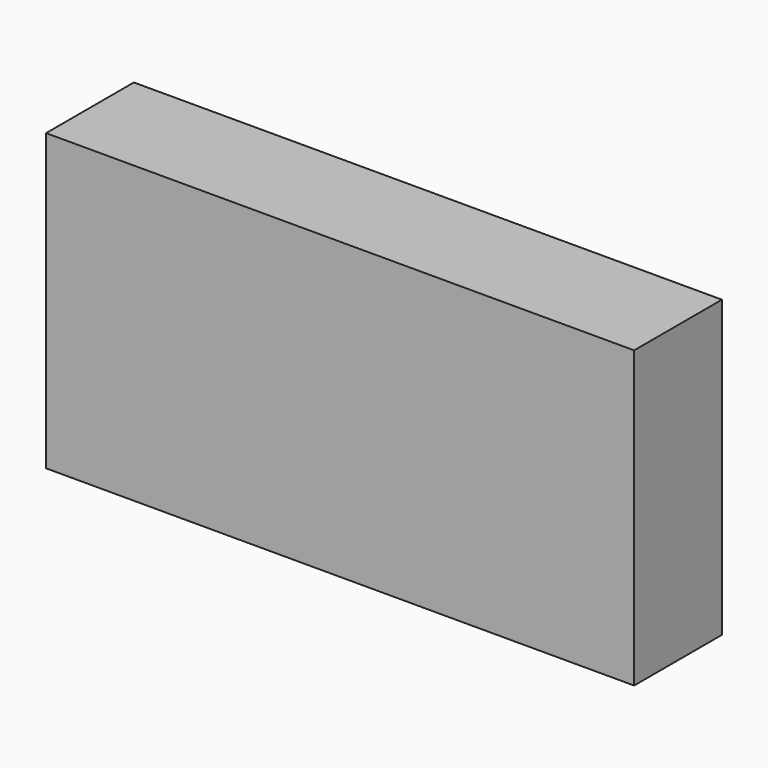
from build123d import *

# Parameters (mm, degrees)
F0_W     = 136.1236646771
F0_H     = 68.3124661446
F1_DEPTH = 25.4


# Not quite as in the source:
# - a feature of the source that left no trace in its solid (it failed there, or was rolled back) is left out


with BuildPart() as f1:
    # F0 (on Front) → F1 (new body)
    with BuildSketch(Plane.XZ):
        with Locations((-12.1615193784, -18.8726782799)):
            Rectangle(F0_W, F0_H)
    extrude(amount=F1_DEPTH)


solid = f1.part
